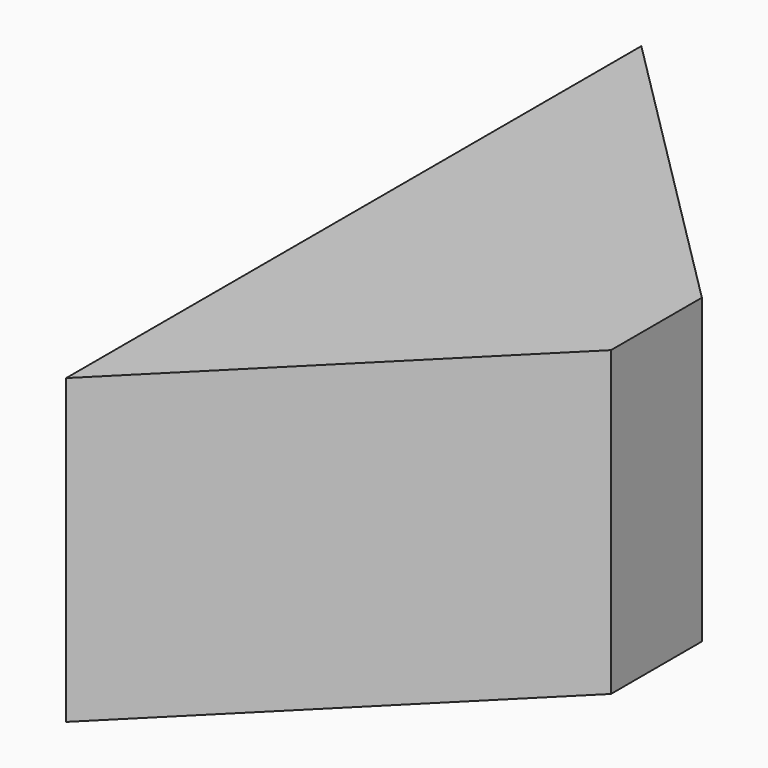
from build123d import *

# Parameters (mm, degrees)
F0_W     = 32.0802
F0_H     = 76.2
F1_DEPTH = 16.0401
F3_DEPTH = 32.0802


# Not quite as in the source:
# - a pattern or mirror of a feature is missing from the dataset's text; its kind, count and spacing are read off the source's solid


with BuildPart() as f1:
    # F0 (on Top) → F1 (new body, symmetric)
    with BuildSketch(Plane.XY):
        Rectangle(F0_W, F0_H)
    extrude(amount=F1_DEPTH, both=True)

    # F2 (on face) → F3 (cut, through all)
    with BuildSketch(Plane.XY.offset(16.0401)):
        Polygon((-16.0401, -38.1), (16.0401, -38.1), (16.0401, -6.0198), align=None)
    f3 = extrude(amount=-F3_DEPTH, mode=Mode.SUBTRACT)

    # F3_copies: F3 across plane
    add(f3.mirror(Plane.ZX), mode=Mode.SUBTRACT)


solid = f1.part
